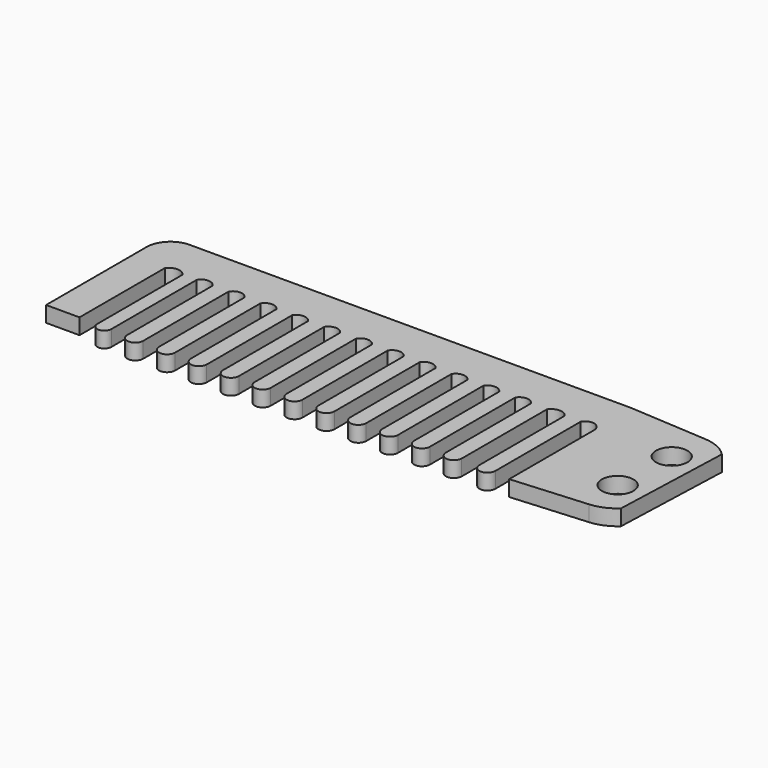
from build123d import *

# Parameters (mm, degrees)
F0_R     = 2
F1_DEPTH = 2


# Not quite as in the source:
# - a feature names something its author has since deleted; it is built from what else it names


with BuildPart() as f1:
    # F0 (on Top) → F1 (new body)
    with BuildSketch(Plane.XY):
        with BuildLine():
            Line((56.6317902379, -3.0349094544), (56.6317902379, 10.5057977874))
            ThreePointArc((56.6317902379, 10.5057977874), (57.9282334063, 11.0612910292), (58.8036425211, 9.955399302))
            Line((58.8036425211, 9.955399302), (58.8036425211, -3.3060063632))
            ThreePointArc((58.8036425211, -3.3060063632), (58.8059571474, -3.4285186947), (58.8128977225, -3.5508561677))
            Line((58.8128977225, -3.5508561677), (68.3904010917, -2.8257703951))
            ThreePointArc((68.3904010917, -2.8257703951), (69.9985927846, -2.4288509841), (71.3888536722, -1.5282954863))
            Line((71.3888536722, -1.5282954863), (71.9441100955, 13.8000454754))
            ThreePointArc((71.9441100955, 13.8000454754), (70.4479915869, 14.8624188349), (68.6693633039, 15.3135165823))
            Line((68.6693633039, 15.3135165823), (58.6544042145, 15.9537835574))
            Line((58.6544042145, 15.9537835574), (2.6067622363, 15.9537835574))
            ThreePointArc((2.6067622363, 15.9537835574), (0.4614561486, 15.0651686804), (-0.4271587284, 12.9198625927))
            Line((-0.4271587284, 12.9198625927), (-0.4271587284, -3.0349094544))
            Line((-0.4271587284, -3.0349094544), (3.8183579072, -3.0349094544))
            Line((3.8183579072, -3.0349094544), (3.8183579072, 2.3688513962))
            Line((3.8183579072, 2.3688513962), (3.8183579072, 10.5057977874))
            ThreePointArc((3.8183579072, 10.5057977874), (4.9481016159, 11.1006888991), (6.0778453246, 10.5057977874))
            Line((6.0778453246, 10.5057977874), (6.0778453246, 2.3688513962))
            Line((6.0778453246, 2.3688513962), (6.0778453246, -3.0349094544))
            ThreePointArc((6.0778453246, -3.0349094544), (6.9707155924, -3.9277797221), (7.8635858601, -3.0349094544))
            Line((7.8635858601, -3.0349094544), (7.8635858601, 2.3688513962))
            Line((7.8635858601, 2.3688513962), (7.8635858601, 10.5057977874))
            ThreePointArc((7.8635858601, 10.5057977874), (8.8748928484, 11.1003156957), (9.8861998366, 10.5057977874))
            Line((9.8861998366, 10.5057977874), (9.8861998366, 2.3688513962))
            Line((9.8861998366, 2.3688513962), (9.8861998366, -3.0349094544))
            ThreePointArc((9.8861998366, -3.0349094544), (10.8975068249, -4.0462164426), (11.9088138131, -3.0349094544))
            Line((11.9088138131, -3.0349094544), (11.9088138131, 2.3688513962))
            Line((11.9088138131, 2.3688513962), (11.9088138131, 10.5057977874))
            ThreePointArc((11.9088138131, 10.5057977874), (12.9201208014, 11.1003953408), (13.9314277896, 10.5057977874))
            Line((13.9314277896, 10.5057977874), (13.9314277896, 2.3688513962))
            Line((13.9314277896, 2.3688513962), (13.9314277896, -3.0349094544))
            ThreePointArc((13.9314277896, -3.0349094544), (14.9427347779, -4.0462164426), (15.9540417661, -3.0349094544))
            Line((15.9540417661, -3.0349094544), (15.9540417661, 2.3688513962))
            Line((15.9540417661, 2.3688513962), (15.9540417661, 10.5057977874))
            ThreePointArc((15.9540417661, 10.5057977874), (16.9653487543, 11.1012729968), (17.9766557426, 10.5057977874))
            Line((17.9766557426, 10.5057977874), (17.9766557426, -3.0349094544))
            Line((17.9766557426, -3.0349094544), (17.9766557426, -3.0600128507))
            ThreePointArc((17.9766557426, -3.0600128507), (18.987884836, -4.0587681408), (19.9991139294, -3.0600128507))
            Line((19.9991139294, -3.0600128507), (19.9991139294, -3.0349094544))
            Line((19.9991139294, -3.0349094544), (19.9991139294, 2.3688513962))
            Line((19.9991139294, 2.3688513962), (19.9991139294, 10.5057977874))
            ThreePointArc((19.9991139294, 10.5057977874), (21.0104988125, 11.0625593301), (22.0218836956, 10.5057977874))
            Line((22.0218836956, 10.5057977874), (22.0218836956, 2.3688513962))
            Line((22.0218836956, 2.3688513962), (22.0218836956, -3.0349094544))
            ThreePointArc((22.0218836956, -3.0349094544), (23.0331906838, -4.0270898738), (24.0444976721, -3.0349094544))
            Line((24.0444976721, -3.0349094544), (24.0444976721, 2.3688513962))
            Line((24.0444976721, 2.3688513962), (24.0444976721, 10.5057977874))
            ThreePointArc((24.0444976721, 10.5057977874), (25.0558046603, 11.1004906415), (26.0671116486, 10.5057977874))
            Line((26.0671116486, 10.5057977874), (26.0671116486, 2.3688513962))
            Line((26.0671116486, 2.3688513962), (26.0671116486, -3.0349094544))
            ThreePointArc((26.0671116486, -3.0349094544), (27.0784186368, -4.0282444578), (28.089725625, -3.0349094544))
            Line((28.089725625, -3.0349094544), (28.089725625, 2.3688513962))
            Line((28.089725625, 2.3688513962), (28.089725625, 10.5057977874))
            ThreePointArc((28.089725625, 10.5057977874), (29.1010326133, 11.1005861122), (30.1123396015, 10.5057977874))
            Line((30.1123396015, 10.5057977874), (30.1123396015, 2.3688513962))
            Line((30.1123396015, 2.3688513962), (30.1123396015, -3.0349094544))
            ThreePointArc((30.1123396015, -3.0349094544), (31.1236465898, -4.0401241658), (32.134953578, -3.0349094544))
            Line((32.134953578, -3.0349094544), (32.134953578, 2.3688513962))
            Line((32.134953578, 2.3688513962), (32.134953578, 10.5057977874))
            ThreePointArc((32.134953578, 10.5057977874), (33.1462605663, 11.0805944093), (34.1575675545, 10.5057977874))
            Line((34.1575675545, 10.5057977874), (34.1575675545, 2.3688513962))
            Line((34.1575675545, 2.3688513962), (34.1575675545, -3.0349094544))
            ThreePointArc((34.1575675545, -3.0349094544), (35.1688745428, -4.0284589293), (36.180181531, -3.0349094544))
            Line((36.180181531, -3.0349094544), (36.180181531, 2.3688513962))
            Line((36.180181531, 2.3688513962), (36.180181531, 10.5057977874))
            ThreePointArc((36.180181531, 10.5057977874), (37.1914885192, 11.0806196167), (38.2027955075, 10.5057977874))
            Line((38.2027955075, 10.5057977874), (38.2027955075, 2.3688513962))
            Line((38.2027955075, 2.3688513962), (38.2027955075, -3.0349094544))
            ThreePointArc((38.2027955075, -3.0349094544), (39.2141024957, -4.0246480782), (40.225409484, -3.0349094544))
            Line((40.225409484, -3.0349094544), (40.225409484, 2.3688513962))
            Line((40.225409484, 2.3688513962), (40.225409484, 10.5057977874))
            ThreePointArc((40.225409484, 10.5057977874), (41.2367164722, 11.0799992786), (42.2480234605, 10.5057977874))
            Line((42.2480234605, 10.5057977874), (42.2480234605, 2.3688513962))
            Line((42.2480234605, 2.3688513962), (42.2480234605, -3.0349094544))
            ThreePointArc((42.2480234605, -3.0349094544), (43.2593304487, -4.0462164426), (44.270637437, -3.0349094544))
            Line((44.270637437, -3.0349094544), (44.270637437, 2.3688513962))
            Line((44.270637437, 2.3688513962), (44.270637437, 10.5057977874))
            ThreePointArc((44.270637437, 10.5057977874), (45.2819444252, 11.0763000676), (46.2932514135, 10.5057977874))
            Line((46.2932514135, 10.5057977874), (46.2932514135, 2.3688513962))
            Line((46.2932514135, 2.3688513962), (46.2932514135, -3.0349094544))
            ThreePointArc((46.2932514135, -3.0349094544), (47.3045584017, -4.0362897846), (48.3158653899, -3.0349094544))
            Line((48.3158653899, -3.0349094544), (48.3158653899, 2.3688513962))
            Line((48.3158653899, 2.3688513962), (48.3158653899, 10.5057977874))
            ThreePointArc((48.3158653899, 10.5057977874), (49.3271723782, 11.0768378201), (50.3384793664, 10.5057977874))
            Line((50.3384793664, 10.5057977874), (50.3384793664, 2.3688513962))
            Line((50.3384793664, 2.3688513962), (50.3384793664, -3.0349094544))
            ThreePointArc((50.3384793664, -3.0349094544), (51.3497863547, -4.0273604844), (52.3610933429, -3.0349094544))
            Line((52.3610933429, -3.0349094544), (52.3610933429, 2.3688513962))
            Line((52.3610933429, 2.3688513962), (52.3610933429, 10.5057977874))
            ThreePointArc((52.3610933429, 10.5057977874), (53.4851541573, 11.0994017223), (54.6092149717, 10.5057977874))
            Line((54.6092149717, 10.5057977874), (54.6092149717, 2.3688513962))
            Line((54.6092149717, 2.3688513962), (54.6092149717, -3.0349094544))
            ThreePointArc((54.6092149717, -3.0349094544), (55.6205026048, -4.039959639), (56.6317902379, -3.0349094544))
        make_face()
        with Locations((68.012945354, 2.1599619649)):
            Circle(F0_R, mode=Mode.SUBTRACT)
        with Locations((68.3503592405, 10.3237033185)):
            Circle(F0_R, mode=Mode.SUBTRACT)
    extrude(amount=F1_DEPTH)


solid = f1.part
